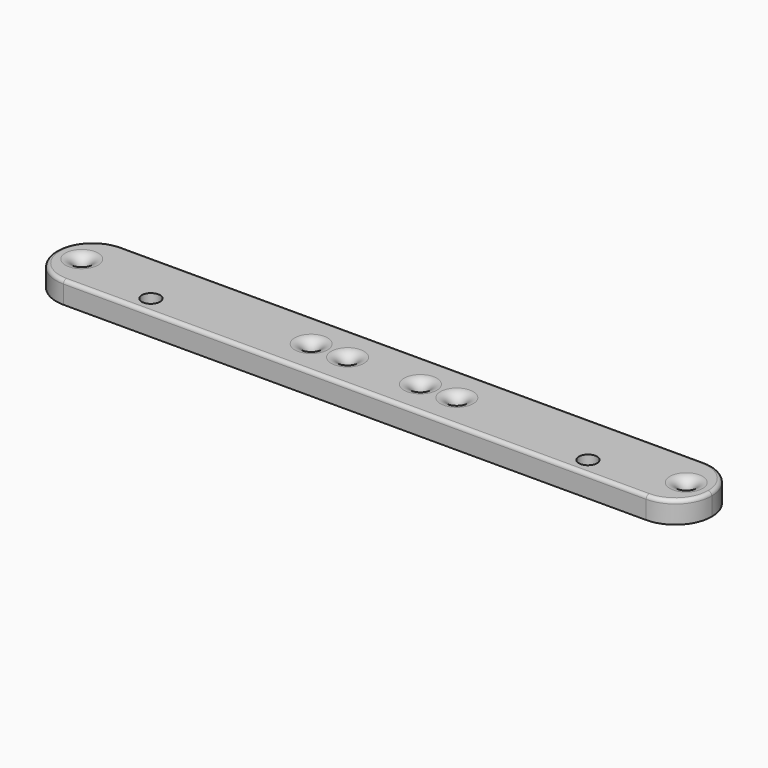
from build123d import *

# Parameters (mm, degrees)
F0_W     = 180
F0_H     = 20
F0_R     = 1.5
F1_DEPTH = 6
F2_R     = 2.99999
F3_R     = 9.99999
F4_W     = 166
F4_H     = 3
F5_DEPTH = 1
F6_R     = 1
F7_R     = 2.5
F8_DEPTH = 25


# Not quite as in the source:
# - a fillet or chamfer is up to 0.001 mm smaller than in the source, because OpenCascade refuses the exact size


with BuildPart() as f1:
    # F0 (on Top) → F1 (new body)
    with BuildSketch(Plane.XY):
        Rectangle(F0_W, F0_H)
        with Locations((-83, 0)):
            Circle(F0_R, mode=Mode.SUBTRACT)
        with Locations((-20, 0)):
            Circle(F0_R, mode=Mode.SUBTRACT)
        with Locations((-10, 0)):
            Circle(F0_R, mode=Mode.SUBTRACT)
        with Locations((10, 0)):
            Circle(F0_R, mode=Mode.SUBTRACT)
        with Locations((20, 0)):
            Circle(F0_R, mode=Mode.SUBTRACT)
        with Locations((83, 0)):
            Circle(F0_R, mode=Mode.SUBTRACT)
    extrude(amount=F1_DEPTH)

    # F2 (radius 3 in the source; OpenCascade refuses exactly that, so slightly less here)
    f2_edges = [f1.edges().sort_by_distance(p)[0] for p in [
        (-84.5, 0, 6),
        (81.5, 0, 6),
        (-84.5, 0, 0),
        (81.5, 0, 0),
        (18.5, 0, 0),
        (8.5, 0, 0),
        (-11.5, 0, 0),
        (-21.5, 0, 0),
        (-21.5, 0, 6),
        (-11.5, 0, 6),
        (8.5, 0, 6),
        (18.5, 0, 6),
    ]]
    fillet(f2_edges, radius=F2_R)

    # F3 (radius 10 in the source; OpenCascade refuses exactly that, so slightly less here)
    f3_edges = [f1.edges().sort_by_distance(p)[0] for p in [
        (-90, -10, 3),
        (-90, 10, 3),
        (90, -10, 3),
        (90, 10, 3),
    ]]
    fillet(f3_edges, radius=F3_R)

    # F4 (on Top) → F5 (cut)
    with BuildSketch(Plane.XY):
        Rectangle(F4_W, F4_H)
    extrude(amount=F5_DEPTH, mode=Mode.SUBTRACT)

    # F6
    f6_edges = [f1.edges().sort_by_distance(p)[0] for p in [
        (0, -10, 6),
    ]]
    fillet(f6_edges, radius=F6_R)

    # F7 (on Top) → F8 (cut)
    with BuildSketch(Plane.XY):
        with Locations((-60, -5)):
            Circle(F7_R)
        with Locations((60, -5)):
            Circle(F7_R)
    extrude(amount=F8_DEPTH, mode=Mode.SUBTRACT)


solid = f1.part
